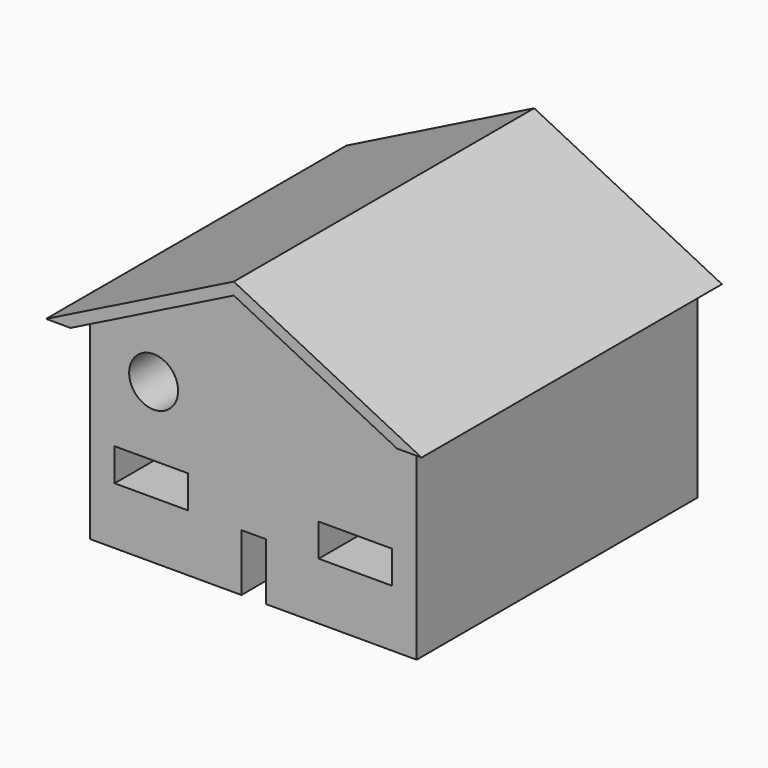
from build123d import *

# Parameters (mm, degrees)
F1_DEPTH = 14020.8
F2_DEPTH = 13106.4
F0_W     = 2743.2
F0_H     = 1219.2
F0_R     = 914.4
F3_DEPTH = 13106.4


# Not quite as in the source:
# - the program builds the solid bodies; features that only make, move or delete a surface that nothing else refers to are left out


with BuildPart() as f1:
    # F0 (on Front) → F1 (new body)
    with BuildSketch(Plane.XZ):
        Polygon((-7010.4, 0), (-6096, 0), (0, 3048), (0, 3505.2), align=None)
        Polygon((0, 3048), (6096, 0), (7010.4, 0), (0, 3505.2), align=None)
    extrude(amount=F1_DEPTH)

    # F0 (on Front) → F2 (join)
    with BuildSketch(Plane.XZ):
        Polygon((-6096, 0), (0, 0), (6096, 0), (0, 3048), align=None)
    extrude(amount=F2_DEPTH)

    # F0 (on Front) → F3 (join)
    with BuildSketch(Plane.XZ):
        Polygon((6096, 0), (0, 0), (-6096, 0), (-6096, -7315.2), (-447.0156319439, -7315.2), (-447.0156319439, -5181.6), (467.3843680561, -5181.6), (467.3843680561, -7315.2), (6096, -7315.2), align=None)
        with Locations((-3810, -4572)):
            Rectangle(F0_W, F0_H, mode=Mode.SUBTRACT)
        with Locations((3810, -4572)):
            Rectangle(F0_W, F0_H, mode=Mode.SUBTRACT)
        with Locations((-3726.0398864746, -1372.2128868103)):
            Circle(F0_R, mode=Mode.SUBTRACT)
    extrude(amount=F3_DEPTH)


solid = f1.part
